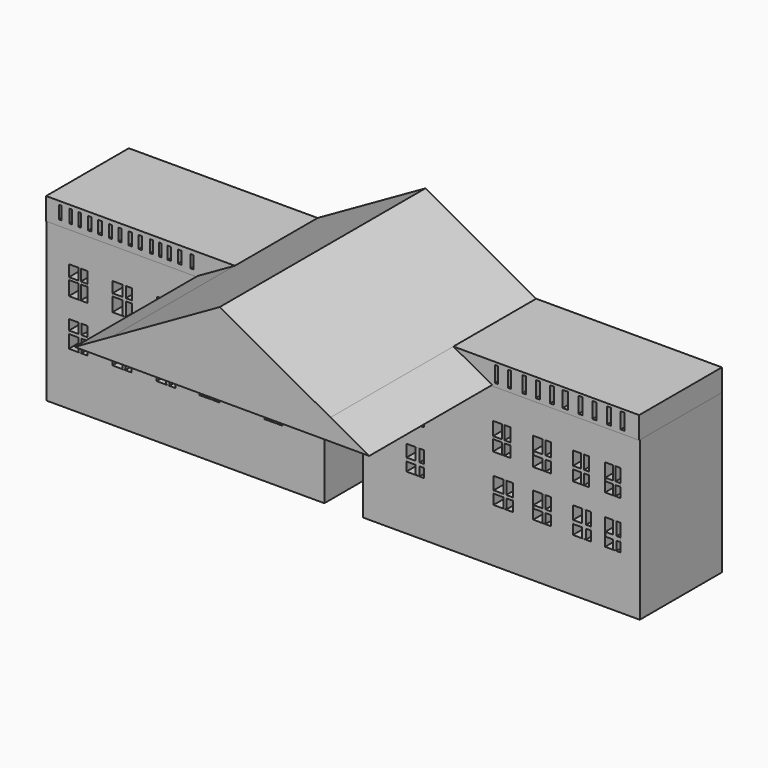
from build123d import *

# Parameters (mm, degrees)
F8_DEPTH  = 35.306
F9_DEPTH  = 88.392
F0_W      = 0.8455142379
F0_H      = 4.5100699443
F0_W_2    = 0.9964480996
F0_H_2    = 4.4677245695
F0_W_3    = 1.0761618614
F0_H_3    = 4.3880070824
F0_W_4    = 1.235589385
F0_H_4    = 4.3082895953
F0_W_5    = 0.956594944
F0_H_5    = 4.2684327144
F0_W_6    = 1.1957362294
F0_W_7    = 1.039005816
F0_W_8    = 0.9716898203
F0_W_9    = 1.1612847447
F0_W_10   = 1.2323819101
F0_W_11   = 1.0054893792
F0_H_6    = 4.3571274728
F0_W_12   = 1.0725222528
F0_H_7    = 5.4966807365
F0_W_13   = 1.340650022
F0_W_14   = 1.4076903462
F0_W_15   = 1.4076828957
F0_W_16   = 1.7428547144
F10_DEPTH = 35.56
F0_W_17   = 0.8613243699
F0_H_8    = 3.9584673941
F0_H_9    = 4.834727617
F0_W_18   = 2.3618265986
F0_H_10   = 0.8762602229
F0_W_19   = 3.2231509686
F0_W_20   = 3.3498592675
F0_H_11   = 0.9820964187
F0_W_21   = 1.0436698794
F0_H_12   = 3.5210016649
F0_H_13   = 1.0767292697
F0_W_22   = 2.1794810891
F0_H_14   = 4.4081346132
F0_W_23   = 1.1096019298
F0_W_24   = 2.9387567192
F0_H_15   = 0.7814618293
F0_W_25   = 1.8291547894
F0_H_16   = 4.7399292234
F0_W_26   = 1.1610034853
F0_W_27   = 3.2231491059
F0_H_17   = 0.9819304105
F0_W_28   = 2.0621456206
F0_H_18   = 4.5029320754
F0_W_29   = 1.2413617224
F0_H_19   = 3.152186051
F0_W_30   = 3.4127477556
F0_H_20   = 1.0754363611
F0_W_31   = 2.1713860333
F0_H_21   = 4.2276224121
F0_W_32   = 0.8478974923
F0_H_22   = 3.768870607
F0_W_33   = 2.5595622137
F0_H_23   = 0.6796028465
F0_W_34   = 1.7116647214
F0_H_24   = 4.4484734535
F0_W_35   = 1.2511014938
F0_W_36   = 3.0335541815
F0_W_37   = 1.7824526876
F0_W_38   = 1.2323815026
F0_H_25   = 4.9270658725
F0_W_39   = 3.0335550546
F0_H_26   = 1.1243226967
F0_W_40   = 1.8011735519
F0_H_27   = 3.8027431758
F0_W_41   = 1.282133162
F0_W_42   = 3.0335523188
F0_W_43   = 1.7514191568
F0_W_44   = 1.5014316887
F0_H_28   = 3.0281706713
F0_H_29   = 1.1994517408
F0_W_45   = 1.5321206301
F0_W_46   = 0.9014569223
F0_H_30   = 4.6451305971
F0_W_47   = 3.0335560441
F0_H_31   = 0.9242631495
F0_W_48   = 2.1320991218
F0_H_32   = 3.7208674476
F0_W_49   = 1.1317506433
F0_W_50   = 3.0709058046
F0_H_33   = 1.2897616252
F0_W_51   = 1.9391551614
F0_H_34   = 3.5449648276
F0_W_52   = 3.3179484308
F0_H_35   = 1.0189395398
F0_W_53   = 1.0122619569
F0_H_36   = 3.3891946077
F0_W_54   = 1.058652997
F0_H_37   = 4.4161728583
F0_H_38   = 1.0840008035
F0_W_55   = 2.0122528076
F0_H_39   = 3.3321720548
F0_W_56   = 1.033551991
F0_H_40   = 4.6851034276
F0_W_57   = 2.7491524816
F0_H_41   = 1.1035888456
F0_W_58   = 1.7156004906
F0_H_42   = 3.581514582
F0_W_59   = 2.6142783463
F0_W_60   = 1.3122521341
F0_H_43   = 4.5029330067
F0_W_61   = 3.1283535063
F0_H_44   = 1.2165401131
F0_H_45   = 3.2863928936
F0_W_62   = 1.8161013722
F0_W_63   = 1.2923441827
F0_H_46   = 1.4358386397
F0_W_64   = 1.3219341636
F0_H_47   = 3.067094367
F0_H_48   = 4.4081341475
F0_W_65   = 2.3056864738
F11_DEPTH = 35.2298
F12_DEPTH = 36.3474


# Not quite as in the source:
# - the program builds the solid bodies; features that only make, move or delete a surface that nothing else refers to are left out


with BuildPart() as f8:
    # F0 (on Front) → F8 (new body)
    with BuildSketch(Plane.XZ):
        with BuildLine():
            Line((-101.9500866532, 27.2123937317), (-101.9500866532, -27.2123937317))
            Line((-101.9500866532, -27.2123937317), (-6.4866924658, -27.2123937317))
            Line((-6.4866924658, -27.2123937317), (-6.4866924658, -7.1731594767))
            ThreePointArc((-6.4866924658, -7.1731594767), (-4.6245261313, -2.3375779185), (0, 0))
            ThreePointArc((0, 0), (4.8074193944, -2.2429274148), (6.7656881291, -7.1731594767))
            Line((6.7656881291, -7.1731594767), (6.7656881291, -27.2123937317))
            Line((6.7656881291, -27.2123937317), (101.9500866532, -27.2123937317))
            Line((101.9500866532, -27.2123937317), (101.9500866532, 27.2123937317))
            Line((101.9500866532, 27.2123937317), (-101.9500866532, 27.2123937317))
        make_face()
        Polygon((-94.3245813251, -3.5210016649), (-94.3245813251, 0), (-91.1014303565, 0), (-90.0577604771, 0), (-87.878279388, 0), (-87.878279388, -3.5210016649), (-87.878279388, -4.5977309346), (-87.878279388, -9.0058655478), (-90.0577604771, -9.0058655478), (-91.1014303565, -9.0058655478), (-94.3245813251, -9.0058655478), (-94.3245813251, -4.5977309346), align=None, mode=Mode.SUBTRACT)
        Polygon((-74.926123023, 0), (-72.6466923952, 0), (-72.6711301256, -3.5210016649), (-72.6786032319, -4.5977309346), (-72.7105140686, -9.1954618692), (-74.926123023, -9.1954618692), (-76.0284624994, -9.1954618692), (-79.3464109302, -9.1954618692), (-79.3464109302, -4.5977309346), (-79.3464109302, -3.5210016649), (-79.3464109302, 0), (-75.9965516627, 0), align=None, mode=Mode.SUBTRACT)
        Polygon((-64.1786381602, -3.5210016649), (-64.1786381602, 0), (-60.9554890543, 0), (-59.794485569, 0), (-57.7323399484, 0), (-57.7323399484, -3.5210016649), (-57.7323399484, -4.5029320754), (-57.7323399484, -9.0058641508), (-59.794485569, -9.0058641508), (-60.9554890543, -9.0058641508), (-64.1786381602, -9.0058641508), (-64.1786381602, -4.5029320754), align=None, mode=Mode.SUBTRACT)
        Polygon((-87.878279388, 11.7550238501), (-87.878279388, 6.9202962331), (-90.2401059866, 6.9202962331), (-91.1014303565, 6.9202962331), (-94.3245813251, 6.9202962331), (-94.3245813251, 11.7550238501), (-94.3245813251, 12.631284073), (-94.3245813251, 16.5897514671), (-91.1014303565, 16.5897514671), (-90.2401059866, 16.5897514671), (-87.878279388, 16.5897514671), (-87.878279388, 12.631284073), align=None, mode=Mode.SUBTRACT)
        Polygon((-74.7800106891, 16.3796447158), (-72.6466923952, 16.3780790754), (-72.6466923952, 12.631284073), (-72.6466923952, 11.6491876543), (-72.6466923952, 6.9202962331), (-74.7869528966, 6.9202962331), (-75.9965516627, 6.9202962331), (-79.3464109302, 6.9202962331), (-79.3464109302, 11.6491876543), (-79.3464109302, 12.631284073), (-79.3464109302, 16.3829959929), (-75.9965516627, 16.3805375341), align=None, mode=Mode.SUBTRACT)
        Polygon((-63.9890432358, 12.631284073), (-63.9890432358, 16.5897514671), (-61.0502865165, 16.5897514671), (-59.9406845868, 16.5897514671), (-58.1115297973, 16.5897514671), (-58.1115297973, 12.631284073), (-58.1115297973, 11.8498222437), (-58.1115297973, 7.1098930202), (-59.9406845868, 7.1098930202), (-61.0502865165, 7.1098930202), (-63.9890432358, 7.1098930202), (-63.9890432358, 11.8498222437), align=None, mode=Mode.SUBTRACT)
        Polygon((-49.3900589645, -3.152186051), (-49.3900589645, 0), (-45.9773112088, 0), (-44.7359494865, 0), (-42.5645634532, 0), (-42.5645634532, -3.152186051), (-42.5645634532, -4.2276224121), (-42.5645634532, -8.4552448243), (-44.7359494865, -8.4552448243), (-45.9773112088, -8.4552448243), (-49.3900589645, -8.4552448243), (-49.3900589645, -4.2276224121), align=None, mode=Mode.SUBTRACT)
        Polygon((-23.984041065, -8.4552448243), (-27.0175952464, -8.4552448243), (-27.0175952464, -4.2276224121), (-27.0175952464, -3.152186051), (-27.0175952464, 0), (-23.984041065, 0), (-22.7329395711, 0), (-20.9504868835, 0), (-20.9504868835, -3.152186051), (-20.9504868835, -4.2276224121), (-20.9504868835, -8.4552448243), (-22.7329395711, -8.4552448243), align=None, mode=Mode.SUBTRACT)
        Polygon((-49.3900589645, 12.631284073), (-49.3900589645, 16.5897514671), (-46.1669079959, 16.5897514671), (-45.1014451683, 16.5897514671), (-42.9437570274, 16.5897514671), (-42.9437570274, 12.631284073), (-42.9437570274, 11.7491195207), (-42.9437570274, 6.9196401976), (-45.1181687338, 6.9234021056), (-46.1669079959, 6.9252165093), (-49.3900589645, 6.9307928209), (-49.3900589645, 11.760272144), align=None, mode=Mode.SUBTRACT)
        Polygon((-24.4580330327, 7.503207773), (-27.0175952464, 7.503207773), (-27.0175952464, 11.9516812265), (-27.0175952464, 12.631284073), (-27.0175952464, 16.40015468), (-24.4580330327, 16.40015468), (-23.6101355404, 16.40015468), (-21.898470819, 16.40015468), (-21.898470819, 12.631284073), (-21.898470819, 11.9516812265), (-21.898470819, 7.503207773), (-23.6101355404, 7.503207773), align=None, mode=Mode.SUBTRACT)
        Polygon((-4.2659365572, 11.8522823817), (-4.2659365572, 16.7793482542), (-1.2323815026, 16.7793482542), (0, 16.7793482542), (1.8011735519, 16.7793482542), (1.8011735519, 11.8522823817), (1.8011735519, 10.727959685), (1.8011735519, 6.9252165093), (0, 6.9252165093), (-1.2323815026, 6.9252165093), (-4.2659365572, 6.9252165093), (-4.2659365572, 10.727959685), align=None, mode=Mode.SUBTRACT)
        Polygon((21.7088758945, -4.2276224121), (21.7088758945, 0), (24.7424282134, 0), (26.243859902, 0), (27.7759805322, 0), (27.7759805322, -4.2276224121), (27.7759805322, -5.427074153), (27.7759805322, -8.4552448243), (26.243859902, -8.4552448243), (24.7424282134, -8.4552448243), (21.7088758945, -8.4552448243), (21.7088758945, -5.427074153), align=None, mode=Mode.SUBTRACT)
        Polygon((21.7088758945, 11.8522823817), (21.7088758945, 16.7793482542), (24.7424282134, 16.7793482542), (26.0245613754, 16.7793482542), (27.7759805322, 16.7793482542), (27.7759805322, 11.8522823817), (27.7759805322, 10.727959685), (27.7759805322, 6.9252165093), (26.0245613754, 6.9252165093), (24.7424282134, 6.9252165093), (21.7088758945, 6.9252165093), (21.7088758945, 10.727959685), align=None, mode=Mode.SUBTRACT)
        Polygon((51.6652278602, -4.4081341475), (51.6652278602, 0), (54.983176291, 0), (55.9954382479, 0), (58.3011247218, 0), (58.3011247218, -4.4081341475), (58.3011247218, -5.4270736873), (58.3011247218, -8.816268295), (55.9954382479, -8.816268295), (54.983176291, -8.816268295), (51.6652278602, -8.816268295), (51.6652278602, -5.4270736873), align=None, mode=Mode.SUBTRACT)
        Polygon((65.3162226081, -4.4161728583), (65.3162226081, 0), (68.3871284127, 0), (69.4457814097, 0), (71.4580342174, 0), (71.4580342174, -4.4161728583), (71.4580342174, -5.5001736619), (71.4580342174, -8.8323457167), (69.4457814097, -8.8323457167), (68.3871284127, -8.8323457167), (65.3162226081, -8.8323457167), (65.3162226081, -5.5001736619), align=None, mode=Mode.SUBTRACT)
        Polygon((78.9672210813, -4.5029330067), (78.9672210813, 0), (82.0955745876, 0), (83.4078267217, 0), (85.2239280939, 0), (85.2239280939, -4.5029330067), (85.2239280939, -5.7194731198), (85.2239280939, -9.0058660135), (83.4078267217, -9.0058660135), (82.0955745876, -9.0058660135), (78.9672210813, -9.0058660135), (78.9672210813, -5.7194731198), align=None, mode=Mode.SUBTRACT)
        Polygon((90.0275558233, -4.5029330067), (90.0275558233, 0), (92.6418341696, 0), (93.9341783524, 0), (95.2561125159, 0), (95.2561125159, -4.5029330067), (95.2561125159, -5.9387716465), (95.2561125159, -9.0058660135), (93.9341783524, -9.0058660135), (92.6418341696, -9.0058660135), (90.0275558233, -9.0058660135), (90.0275558233, -5.9387716465), align=None, mode=Mode.SUBTRACT)
        Polygon((51.4756254852, 11.9446208701), (51.4756254852, 16.5897514671), (54.5091815293, 16.5897514671), (55.4106384516, 16.5897514671), (57.5427375734, 16.5897514671), (57.5427375734, 11.9446208701), (57.5427375734, 11.0203577206), (57.5427375734, 7.299490273), (55.4106384516, 7.299490273), (54.5091815293, 7.299490273), (51.4756254852, 7.299490273), (51.4756254852, 11.0203577206), align=None, mode=Mode.SUBTRACT)
        Polygon((65.3162226081, 11.9446208701), (65.3162226081, 16.5897514671), (68.3871284127, 16.5897514671), (69.518879056, 16.5897514671), (71.4580342174, 16.5897514671), (71.4580342174, 11.9446208701), (71.4580342174, 10.6548592448), (71.4580342174, 7.1098944172), (69.518879056, 7.1098944172), (68.3871284127, 7.1098944172), (65.3162226081, 7.1098944172), (65.3162226081, 10.6548592448), align=None, mode=Mode.SUBTRACT)
        Polygon((78.9672210813, 11.9046480395), (78.9672210813, 16.5897514671), (81.7163735628, 16.5897514671), (82.7499255538, 16.5897514671), (84.4655260444, 16.5897514671), (84.4655260444, 11.9046480395), (84.4655260444, 10.8010591939), (84.4655260444, 7.2195446119), (82.7499255538, 7.2195446119), (81.7163735628, 7.2195446119), (78.9672210813, 7.2195446119), (78.9672210813, 10.8010591939), align=None, mode=Mode.SUBTRACT)
        Polygon((90.0275558233, 11.9046480395), (90.0275558233, 16.5897514671), (92.6418341696, 16.5897514671), (93.4995114803, 16.5897514671), (95.2561125159, 16.5897514671), (95.2561125159, 11.9046480395), (95.2561125159, 10.8010591939), (95.2561125159, 7.4473102577), (93.5985073447, 7.4473102577), (92.6418341696, 7.4473102577), (90.0275558233, 7.4473102577), (90.0275558233, 10.8010591939), align=None, mode=Mode.SUBTRACT)
    extrude(amount=F8_DEPTH)

    # F0 (on Front) → F11 (join)
    with BuildSketch(Plane.XZ):
        with Locations((-90.6707681715, 14.6105177701)):
            Rectangle(F0_W_17, F0_H_8)
        with Locations((-90.6707681715, 9.3376600416)):
            Rectangle(F0_W_17, F0_H_9)
        with Locations((-89.0591926873, 12.1931539616)):
            Rectangle(F0_W_18, F0_H_10)
        with Locations((-92.7130058408, 12.1931539616)):
            Rectangle(F0_W_19, F0_H_10)
        Polygon((-74.7827616077, 12.631284073), (-74.7800106891, 16.3796447158), (-75.9965516627, 16.3805375341), (-75.9965516627, 12.631284073), align=None)
        with Locations((-77.6714812964, 12.1402358636)):
            Rectangle(F0_W_20, F0_H_11)
        Polygon((-72.6466923952, 11.6491876543), (-72.6466923952, 12.631284073), (-74.7827616077, 12.631284073), (-74.7834823674, 11.6491876543), align=None)
        Polygon((-74.7869528966, 6.9202962331), (-74.7834823674, 11.6491876543), (-75.9965516627, 11.6491876543), (-75.9965516627, 6.9202962331), align=None)
        with Locations((-90.5795954168, -1.7605008325)):
            Rectangle(F0_W_21, F0_H_12)
        with Locations((-92.7130058408, -4.0593662998)):
            Rectangle(F0_W_19, F0_H_13)
        with Locations((-88.9680199325, -4.0593662998)):
            Rectangle(F0_W_22, F0_H_13)
        with Locations((-90.5795954168, -6.8017982412)):
            Rectangle(F0_W_21, F0_H_14)
        Polygon((-74.926123023, -3.5210016649), (-74.926123023, 0), (-75.9965516627, 0), (-76.0087705279, -3.5210016649), align=None)
        Polygon((-76.012507081, -4.5977309346), (-76.0087705279, -3.5210016649), (-79.3464109302, -3.5210016649), (-79.3464109302, -4.5977309346), align=None)
        Polygon((-72.6786032319, -4.5977309346), (-72.6711301256, -3.5210016649), (-74.926123023, -3.5210016649), (-74.926123023, -4.5977309346), align=None)
        Polygon((-74.926123023, -9.1954618692), (-74.926123023, -4.5977309346), (-76.012507081, -4.5977309346), (-76.0284624994, -9.1954618692), align=None)
        with Locations((-60.4954855517, 14.6105177701)):
            Rectangle(F0_W_23, F0_H_8)
        with Locations((-62.5196648762, 12.2405531583)):
            Rectangle(F0_W_24, F0_H_15)
        with Locations((-59.026107192, 12.2405531583)):
            Rectangle(F0_W_25, F0_H_15)
        with Locations((-60.4954855517, 9.479857632)):
            Rectangle(F0_W_23, F0_H_16)
        Polygon((-45.1014451683, 16.5897514671), (-46.1669079959, 16.5897514671), (-46.1669079959, 12.631284073), (-45.1082936367, 12.631284073), align=None)
        Polygon((-45.1098133693, 11.7528669732), (-46.1669079959, 11.7546958324), (-46.1669079959, 6.9252165093), (-45.1181687338, 6.9234021056), align=None)
        Polygon((-42.9437570274, 12.631284073), (-45.1082936367, 12.631284073), (-45.1098133693, 11.7528669732), (-42.9437570274, 11.7491195207), align=None)
        with Locations((-60.4954855517, 12.2405531583)):
            Rectangle(F0_W_23, F0_H_15)
        Polygon((-46.1669079959, 12.631284073), (-49.3900589645, 12.631284073), (-49.3900589645, 11.760272144), (-46.1669079959, 11.7546958324), align=None)
        Polygon((-45.1082936367, 12.631284073), (-46.1669079959, 12.631284073), (-46.1669079959, 11.7546958324), (-45.1098133693, 11.7528669732), align=None)
        Polygon((-74.7834823674, 11.6491876543), (-74.7827616077, 12.631284073), (-75.9965516627, 12.631284073), (-75.9965516627, 11.6491876543), align=None)
        with Locations((-90.6707681715, 12.1931539616)):
            Rectangle(F0_W_17, F0_H_10)
        with Locations((-90.5795954168, -4.0593662998)):
            Rectangle(F0_W_21, F0_H_13)
        Polygon((-74.926123023, -4.5977309346), (-74.926123023, -3.5210016649), (-76.0087705279, -3.5210016649), (-76.012507081, -4.5977309346), align=None)
        with Locations((-60.3749873117, -1.7605008325)):
            Rectangle(F0_W_26, F0_H_12)
        with Locations((-62.5670636073, -4.0119668702)):
            Rectangle(F0_W_27, F0_H_17)
        with Locations((-58.7634127587, -4.0119668702)):
            Rectangle(F0_W_28, F0_H_17)
        with Locations((-60.3749873117, -6.7543981131)):
            Rectangle(F0_W_26, F0_H_18)
        with Locations((-60.3749873117, -4.0119668702)):
            Rectangle(F0_W_26, F0_H_17)
        with Locations((-45.3566303477, -1.5760930255)):
            Rectangle(F0_W_29, F0_H_19)
        with Locations((-47.6836850867, -3.6899042316)):
            Rectangle(F0_W_30, F0_H_20)
        with Locations((-43.6502564698, -3.6899042316)):
            Rectangle(F0_W_31, F0_H_20)
        with Locations((-45.3566303477, -6.3414336182)):
            Rectangle(F0_W_29, F0_H_21)
        with Locations((-45.3566303477, -3.6899042316)):
            Rectangle(F0_W_29, F0_H_20)
        with Locations((-24.0340842865, 14.5157193765)):
            Rectangle(F0_W_32, F0_H_22)
        with Locations((-25.7378141396, 12.2914826497)):
            Rectangle(F0_W_33, F0_H_23)
        with Locations((-24.0340842865, 12.2914826497)):
            Rectangle(F0_W_32, F0_H_23)
        with Locations((-22.7543031797, 12.2914826497)):
            Rectangle(F0_W_34, F0_H_23)
        with Locations((-24.0340842865, 9.7274444997)):
            Rectangle(F0_W_32, F0_H_24)
        with Locations((-23.3584903181, -1.5760930255)):
            Rectangle(F0_W_35, F0_H_19)
        with Locations((-25.5008181557, -3.6899042316)):
            Rectangle(F0_W_36, F0_H_20)
        with Locations((-23.3584903181, -3.6899042316)):
            Rectangle(F0_W_35, F0_H_20)
        with Locations((-21.8417132273, -3.6899042316)):
            Rectangle(F0_W_37, F0_H_20)
        with Locations((-23.3584903181, -6.3414336182)):
            Rectangle(F0_W_35, F0_H_21)
        with Locations((-0.6161907513, 14.315815318)):
            Rectangle(F0_W_38, F0_H_25)
        with Locations((-2.7491590299, 11.2901210334)):
            Rectangle(F0_W_39, F0_H_26)
        with Locations((-0.6161907513, 11.2901210334)):
            Rectangle(F0_W_38, F0_H_26)
        with Locations((0.900586776, 11.2901210334)):
            Rectangle(F0_W_40, F0_H_26)
        with Locations((-0.6161907513, 8.8265880971)):
            Rectangle(F0_W_38, F0_H_27)
        with Locations((25.3834947944, 14.315815318)):
            Rectangle(F0_W_41, F0_H_25)
        with Locations((25.3834947944, 11.2901210334)):
            Rectangle(F0_W_41, F0_H_26)
        with Locations((25.3834947944, 8.8265880971)):
            Rectangle(F0_W_41, F0_H_27)
        with Locations((23.225652054, 11.2901210334)):
            Rectangle(F0_W_42, F0_H_26)
        with Locations((26.9002709538, 11.2901210334)):
            Rectangle(F0_W_43, F0_H_26)
        with Locations((25.4931440577, -2.1138112061)):
            Rectangle(F0_W_44, F0_H_21)
        with Locations((25.4931440577, -6.9411594886)):
            Rectangle(F0_W_44, F0_H_28)
        with Locations((23.225652054, -4.8273482826)):
            Rectangle(F0_W_42, F0_H_29)
        with Locations((27.0099202171, -4.8273482826)):
            Rectangle(F0_W_45, F0_H_29)
        with Locations((25.4931440577, -4.8273482826)):
            Rectangle(F0_W_44, F0_H_29)
        with Locations((54.9599099904, 14.2671861686)):
            Rectangle(F0_W_46, F0_H_30)
        with Locations((52.9924035072, 11.4824892953)):
            Rectangle(F0_W_47, F0_H_31)
        with Locations((56.4766880125, 11.4824892953)):
            Rectangle(F0_W_48, F0_H_31)
        with Locations((54.9599099904, 9.1599239968)):
            Rectangle(F0_W_46, F0_H_32)
        with Locations((54.9599099904, 11.4824892953)):
            Rectangle(F0_W_46, F0_H_31)
        with Locations((68.9530037344, 14.2671861686)):
            Rectangle(F0_W_49, F0_H_30)
        with Locations((66.8516755104, 11.2997400574)):
            Rectangle(F0_W_50, F0_H_33)
        with Locations((70.4884566367, 11.2997400574)):
            Rectangle(F0_W_51, F0_H_33)
        with Locations((68.9530037344, 8.882376831)):
            Rectangle(F0_W_49, F0_H_34)
        with Locations((68.9530037344, 11.2997400574)):
            Rectangle(F0_W_49, F0_H_33)
        with Locations((53.3242020756, -4.9176039174)):
            Rectangle(F0_W_52, F0_H_35)
        with Locations((55.4893072695, -7.1216709912)):
            Rectangle(F0_W_53, F0_H_36)
        with Locations((68.9164549112, -2.2080864292)):
            Rectangle(F0_W_54, F0_H_37)
        with Locations((66.8516755104, -4.9581732601)):
            Rectangle(F0_W_50, F0_H_38)
        with Locations((68.9164549112, -4.9581732601)):
            Rectangle(F0_W_54, F0_H_38)
        with Locations((70.4519078135, -4.9581732601)):
            Rectangle(F0_W_55, F0_H_38)
        with Locations((68.9164549112, -7.1662596893)):
            Rectangle(F0_W_54, F0_H_39)
        with Locations((82.2331495583, 14.2471997533)):
            Rectangle(F0_W_56, F0_H_40)
        with Locations((80.341797322, 11.3528536167)):
            Rectangle(F0_W_57, F0_H_41)
        with Locations((83.6077257991, 11.3528536167)):
            Rectangle(F0_W_58, F0_H_41)
        with Locations((82.2331495583, 9.0103019029)):
            Rectangle(F0_W_56, F0_H_42)
        with Locations((82.2331495583, 11.3528536167)):
            Rectangle(F0_W_56, F0_H_41)
        Polygon((93.4995114803, 16.5897514671), (92.6418341696, 16.5897514671), (92.6418341696, 11.9046480395), (93.5502425546, 11.9046480395), align=None)
        with Locations((91.3346949965, 11.3528536167)):
            Rectangle(F0_W_59, F0_H_41)
        Polygon((93.5502425546, 11.9046480395), (92.6418341696, 11.9046480395), (92.6418341696, 10.8010591939), (93.562192397, 10.8010591939), align=None)
        Polygon((95.2561125159, 11.9046480395), (93.5502425546, 11.9046480395), (93.562192397, 10.8010591939), (95.2561125159, 10.8010591939), align=None)
        Polygon((93.562192397, 10.8010591939), (92.6418341696, 10.8010591939), (92.6418341696, 7.4473102577), (93.5985073447, 7.4473102577), align=None)
        with Locations((82.7517006546, -2.2514665034)):
            Rectangle(F0_W_60, F0_H_43)
        with Locations((80.5313978344, -5.1112030633)):
            Rectangle(F0_W_61, F0_H_44)
        with Locations((82.7517006546, -7.3626695666)):
            Rectangle(F0_W_60, F0_H_45)
        with Locations((84.3158774078, -5.1112030633)):
            Rectangle(F0_W_62, F0_H_44)
        with Locations((82.7517006546, -5.1112030633)):
            Rectangle(F0_W_60, F0_H_44)
        with Locations((93.288006261, -2.2514665034)):
            Rectangle(F0_W_63, F0_H_43)
        with Locations((91.3346949965, -5.2208523266)):
            Rectangle(F0_W_59, F0_H_46)
        with Locations((93.288006261, -5.2208523266)):
            Rectangle(F0_W_63, F0_H_46)
        with Locations((94.5951454341, -5.2208523266)):
            Rectangle(F0_W_64, F0_H_46)
        with Locations((93.288006261, -7.47231883)):
            Rectangle(F0_W_63, F0_H_47)
        with Locations((55.4893072695, -2.2040670738)):
            Rectangle(F0_W_53, F0_H_48)
        with Locations((57.1482814848, -4.9176039174)):
            Rectangle(F0_W_65, F0_H_35)
        with Locations((55.4893072695, -4.9176039174)):
            Rectangle(F0_W_53, F0_H_35)
    extrude(amount=F11_DEPTH)

    # F0 (on Front) → F12 (join)
    with BuildSketch(Plane.XZ):
        with BuildLine():
            ThreePointArc((0, 0), (-4.6245261313, -2.3375779185), (-6.4866924658, -7.1731594767))
            Line((-6.4866924658, -7.1731594767), (6.7656881291, -7.1731594767))
            ThreePointArc((6.7656881291, -7.1731594767), (4.8074193944, -2.2429274148), (0, 0))
        make_face()
    extrude(amount=F12_DEPTH)


with BuildPart() as f9:
    # F0 (on Front) → F9 (new body)
    with BuildSketch(Plane.XZ):
        Polygon((0, 55.8502785861), (-37.0466325436, 34.8398052156), (-49.8453192413, 27.5812111795), (51.3931550086, 27.5056995451), (38.0952743441, 34.8398052156), align=None)
    extrude(amount=F9_DEPTH)


with BuildPart() as f10:
    # F0 (on Front) → F10 (new body)
    with BuildSketch(Plane.XZ):
        Polygon((-101.9500866532, 34.8398052156), (-101.9500866532, 27.2123937317), (101.9500866532, 27.2123937317), (101.9500866532, 34.8398052156), (38.0952743441, 34.8398052156), (51.3931550086, 27.5056995451), (-49.8453192413, 27.5812111795), (-37.0466325436, 34.8398052156), align=None)
        Polygon((-97.5856930017, 29.1393361986), (-97.5856930017, 33.6487442255), (-96.6837742395, 33.6487442255), (-96.6837742395, 29.1386742812), align=None, mode=Mode.SUBTRACT)
        with Locations((-93.499045819, 31.3937092533)):
            Rectangle(F0_W, F0_H, mode=Mode.SUBTRACT)
        with Locations((-90.3895460069, 31.3725365659)):
            Rectangle(F0_W_2, F0_H_2, mode=Mode.SUBTRACT)
        with Locations((-86.9219079614, 31.3326778224)):
            Rectangle(F0_W_3, F0_H_3, mode=Mode.SUBTRACT)
        with Locations((-83.4144130349, 31.2928190788)):
            Rectangle(F0_W_4, F0_H_4, mode=Mode.SUBTRACT)
        with Locations((-79.8072740436, 31.2728906384)):
            Rectangle(F0_W_5, F0_H_5, mode=Mode.SUBTRACT)
        with Locations((-76.5389241278, 31.2728906384)):
            Rectangle(F0_W_6, F0_H_5, mode=Mode.SUBTRACT)
        with Locations((-73.0712898076, 31.2728906384)):
            Rectangle(F0_W_6, F0_H_5, mode=Mode.SUBTRACT)
        with Locations((-69.5239417255, 31.2728906384)):
            Rectangle(F0_W_6, F0_H_5, mode=Mode.SUBTRACT)
        with Locations((-65.7679475844, 31.2728906384)):
            Rectangle(F0_W_7, F0_H_5, mode=Mode.SUBTRACT)
        with Locations((-62.6832023263, 31.2728906384)):
            Rectangle(F0_W_8, F0_H_5, mode=Mode.SUBTRACT)
        with Locations((-59.55484882, 31.2728906384)):
            Rectangle(F0_W_9, F0_H_5, mode=Mode.SUBTRACT)
        with Locations((-55.9880528599, 31.2728906384)):
            Rectangle(F0_W_10, F0_H_5, mode=Mode.SUBTRACT)
        with Locations((-51.8073830754, 31.2718609348)):
            Rectangle(F0_W_11, F0_H_6, mode=Mode.SUBTRACT)
        with Locations((52.8642069548, 31.171310693)):
            Rectangle(F0_W_12, F0_H_7, mode=Mode.SUBTRACT)
        with Locations((57.4224311858, 31.171310693)):
            Rectangle(F0_W_12, F0_H_7, mode=Mode.SUBTRACT)
        with Locations((62.4498836696, 31.171310693)):
            Rectangle(F0_W_13, F0_H_7, mode=Mode.SUBTRACT)
        with Locations((67.1086572111, 31.171310693)):
            Rectangle(F0_W_14, F0_H_7, mode=Mode.SUBTRACT)
        with Locations((72.0020458102, 31.171310693)):
            Rectangle(F0_W_15, F0_H_7, mode=Mode.SUBTRACT)
        with Locations((76.5267536044, 31.171310693)):
            Rectangle(F0_W_16, F0_H_7, mode=Mode.SUBTRACT)
        with Locations((81.7217901349, 31.171310693)):
            Rectangle(F0_W_15, F0_H_7, mode=Mode.SUBTRACT)
        with Locations((86.5481421351, 31.171310693)):
            Rectangle(F0_W_15, F0_H_7, mode=Mode.SUBTRACT)
        with Locations((91.5756002069, 31.171310693)):
            Rectangle(F0_W_15, F0_H_7, mode=Mode.SUBTRACT)
        with Locations((96.2678864598, 31.171310693)):
            Rectangle(F0_W_15, F0_H_7, mode=Mode.SUBTRACT)
    extrude(amount=F10_DEPTH)


solid = Compound([f8.part, f9.part, f10.part])
